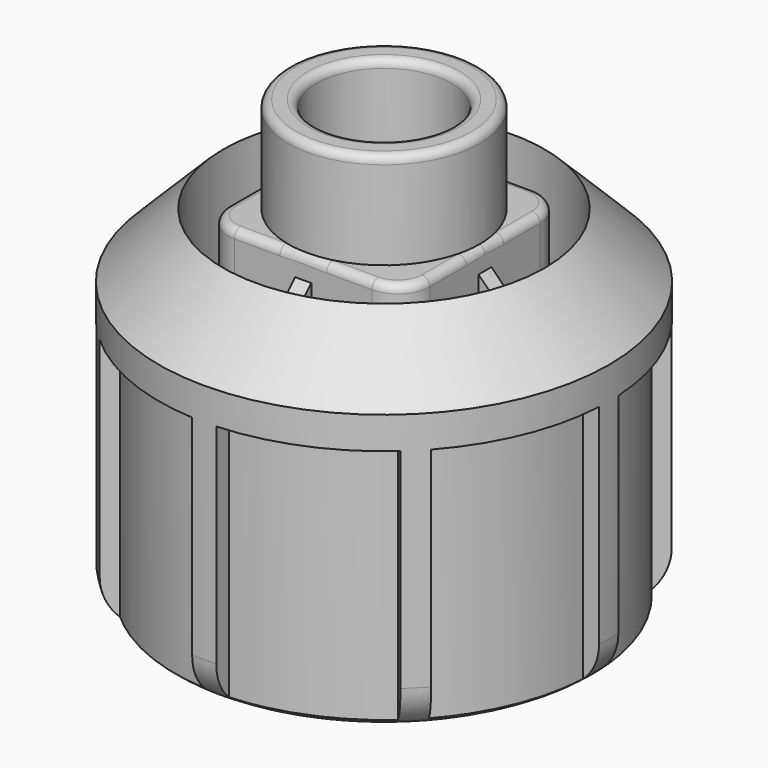
from build123d import *

# Parameters (mm, degrees)
F0_R          = 9.4615
F0_R_2        = 5.08
F1_DEPTH      = 44.45
F2_R          = 22.225
F2_R_2        = 5.08
F3_DEPTH      = 34.925
F4_R          = 6.6675
F5_DEPTH      = 8.128
F6_W          = 13.208
F6_H          = 13.208
F1_FACE1_R    = 9.4615
F1_FACE1_R_2  = 6.6675
F7_DEPTH      = 33.528
F8_R          = 15.875
F9_DEPTH      = 11.684
F10_W         = 3.175
F10_H         = 1.5875
F10_W_2       = 1.5875
F10_H_2       = 3.175
F11_DEPTH     = 9.525
F12_SIZE      = 3.17499
F14_DEPTH     = 25.4
F15_T2_ANGLE  = 33.7650687585
F15_T4_ANGLE  = 33.7650687585
F15_T6_ANGLE  = 67.5302236242
F15_T8_ANGLE  = 67.5302236242
F15_T10_ANGLE = 67.5302236242
F15_T12_ANGLE = 67.5302236242
F15_T14_ANGLE = 67.5302236242
F15_T16_ANGLE = 67.5302236242
F15_T18_ANGLE = 67.5302236242
F16_SIZE      = 6.34999
F17_R         = 0.79375


# Not quite as in the source:
# - a fillet or chamfer that OpenCascade refuses, or shapes differently, is made with other operations: its cross-section is extruded or revolved along the edge and cut away or added
# - a fillet or chamfer is up to 0.001 mm smaller than in the source, because OpenCascade refuses the exact size


with BuildPart() as f1:
    # F0 (on Top) → F1 (new body)
    with BuildSketch(Plane.XY):
        Circle(F0_R)
        Circle(F0_R_2, mode=Mode.SUBTRACT)
    extrude(amount=F1_DEPTH)

    # F2 (on face) → F3 (join)
    with BuildSketch(Plane(origin=(0, 0, 0), x_dir=(1, 0, 0), z_dir=(0, 0, -1))):
        Circle(F2_R)
        Circle(F2_R_2, mode=Mode.SUBTRACT)
    extrude(amount=-F3_DEPTH)

    # F4 (on face) → F5 (cut)
    with BuildSketch(Plane.XY.offset(44.45)):
        Circle(F4_R)
    extrude(amount=-F5_DEPTH, mode=Mode.SUBTRACT)

    # F6 (on face) + F1_face1 (on face) → F7 (cut)
    with BuildSketch(Plane(origin=(0, 0, 0), x_dir=(1, 0, 0), z_dir=(0, 0, -1))):
        Rectangle(F6_W, F6_H)
    with BuildSketch(Plane.XY.offset(44.45)):
        Circle(F1_FACE1_R)
        Circle(F1_FACE1_R_2, mode=Mode.SUBTRACT)
    extrude(amount=-F7_DEPTH, dir=(0, 0, -1), mode=Mode.SUBTRACT)

    # F8 (on face) → F9 (cut)
    with BuildSketch(Plane.XY.offset(34.925)):
        Circle(F8_R)
        with BuildLine():
            Line((-6.7945, 9.9695), (6.7945, 9.9695))
            ThreePointArc((6.7945, 9.9695), (9.0395640303, 9.0395640303), (9.9695, 6.7945))
            Line((9.9695, 6.7945), (9.9695, -6.7945))
            ThreePointArc((9.9695, -6.7945), (9.0395640303, -9.0395640303), (6.7945, -9.9695))
            Line((6.7945, -9.9695), (-6.7945, -9.9695))
            ThreePointArc((-6.7945, -9.9695), (-9.0395640303, -9.0395640303), (-9.9695, -6.7945))
            Line((-9.9695, -6.7945), (-9.9695, 6.7945))
            ThreePointArc((-9.9695, 6.7945), (-9.0395640303, 9.0395640303), (-6.7945, 9.9695))
        make_face(mode=Mode.SUBTRACT)
    extrude(amount=-F9_DEPTH, mode=Mode.SUBTRACT)

    # F10 (on face) → F11 (join)
    with BuildSketch(Plane.XY.offset(23.241)):
        with Locations((-11.557, 0)):
            Rectangle(F10_W, F10_H)
        with Locations((0, -11.557)):
            Rectangle(F10_W_2, F10_H_2)
        with Locations((11.557, 0)):
            Rectangle(F10_W, F10_H)
        with Locations((0, 11.557)):
            Rectangle(F10_W_2, F10_H_2)
    extrude(amount=F11_DEPTH)

    # F12 (size 3.175 in the source; OpenCascade refuses exactly that, so slightly less here)
    f12_edges = [f1.edges().sort_by_distance(p)[0] for p in [
        (-13.1445, 0, 32.766),
        (0, -13.1445, 32.766),
        (13.1445, 0, 32.766),
        (0, 13.1445, 32.766),
    ]]
    chamfer(f12_edges, length=F12_SIZE)

    # F13 (on face) → F14 (cut)
    with BuildSketch(Plane(origin=(0, 0, 0), x_dir=(1, 0, 0), z_dir=(0, 0, -1))):
        with BuildLine():
            Line((22.1930853445, -1.190625), (20.603126422, -1.190625))
            ThreePointArc((20.603126422, -1.190625), (19.0665638522, -7.8976293354), (15.410509418, -13.7267113953))
            Line((15.410509418, -13.7267113953), (16.5347801539, -14.8509821312))
            ThreePointArc((16.5347801539, -14.8509821312), (20.5332226101, -8.5051392843), (22.1930853445, -1.190625))
        make_face()
        with BuildLine():
            Line((14.8509821312, -16.5347801539), (13.7267113953, -15.410509418))
            ThreePointArc((13.7267113953, -15.410509418), (7.8976293354, -19.0665638522), (1.190625, -20.603126422))
            Line((1.190625, -20.603126422), (1.190625, -22.1930853445))
            ThreePointArc((1.190625, -22.1930853445), (8.5051392843, -20.5332226101), (14.8509821312, -16.5347801539))
        make_face()
        with BuildLine():
            Line((-1.190625, -22.1930853445), (-1.190625, -20.603126422))
            ThreePointArc((-1.190625, -20.603126422), (-7.8976293354, -19.0665638522), (-13.7267113953, -15.410509418))
            Line((-13.7267113953, -15.410509418), (-14.8509821312, -16.5347801539))
            ThreePointArc((-14.8509821312, -16.5347801539), (-8.5051392843, -20.5332226101), (-1.190625, -22.1930853445))
        make_face()
        with BuildLine():
            Line((-16.5347801539, -14.8509821312), (-15.410509418, -13.7267113953))
            ThreePointArc((-15.410509418, -13.7267113953), (-19.0665638522, -7.8976293354), (-20.603126422, -1.190625))
            Line((-20.603126422, -1.190625), (-22.1930853445, -1.190625))
            ThreePointArc((-22.1930853445, -1.190625), (-20.5332226101, -8.5051392843), (-16.5347801539, -14.8509821312))
        make_face()
        with BuildLine():
            ThreePointArc((-20.603126422, 1.190625), (-19.0665638522, 7.8976293354), (-15.410509418, 13.7267113953))
            Line((-15.410509418, 13.7267113953), (-16.5347801539, 14.8509821312))
            ThreePointArc((-16.5347801539, 14.8509821312), (-20.5332226101, 8.5051392843), (-22.1930853445, 1.190625))
            Line((-22.1930853445, 1.190625), (-20.603126422, 1.190625))
        make_face()
        with BuildLine():
            ThreePointArc((-13.7267113953, 15.410509418), (-7.8976293354, 19.0665638522), (-1.190625, 20.603126422))
            Line((-1.190625, 20.603126422), (-1.190625, 22.1930853445))
            ThreePointArc((-1.190625, 22.1930853445), (-8.5051392843, 20.5332226101), (-14.8509821312, 16.5347801539))
            Line((-14.8509821312, 16.5347801539), (-13.7267113953, 15.410509418))
        make_face()
        with BuildLine():
            ThreePointArc((1.190625, 20.603126422), (7.8976293354, 19.0665638522), (13.7267113953, 15.410509418))
            Line((13.7267113953, 15.410509418), (14.8509821312, 16.5347801539))
            ThreePointArc((14.8509821312, 16.5347801539), (8.5051392843, 20.5332226101), (1.190625, 22.1930853445))
            Line((1.190625, 22.1930853445), (1.190625, 20.603126422))
        make_face()
        with BuildLine():
            ThreePointArc((15.410509418, 13.7267113953), (19.0665638522, 7.8976293354), (20.603126422, 1.190625))
            Line((20.603126422, 1.190625), (22.1930853445, 1.190625))
            ThreePointArc((22.1930853445, 1.190625), (20.5332226101, 8.5051392843), (16.5347801539, 14.8509821312))
            Line((16.5347801539, 14.8509821312), (15.410509418, 13.7267113953))
        make_face()
    extrude(amount=-F14_DEPTH, mode=Mode.SUBTRACT)

    # F15: fillet of radius 4.7625 on 9 edges, made by hand

    # F15_s1 → F15_t2 (revolve, cut)
    with BuildSketch(Plane(origin=(0, 0, 0), x_dir=(0, 0, 1), z_dir=(-0.5557888899, 0.8313234689, 0))):
        with BuildLine():
            ThreePointArc((4.7625, 22.225), (1.3949039546, 20.8300960454), (0, 17.4625))
            Line((0, 17.4625), (0, 22.225))
            Line((0, 22.225), (4.7625, 22.225))
        make_face()
    revolve(axis=Axis((0, 0, 0), (0, 0, -1)), revolution_arc=F15_T2_ANGLE, mode=Mode.SUBTRACT)

    # F15_s3 → F15_t4 (revolve, cut)
    with BuildSketch(Plane.XZ):
        with BuildLine():
            ThreePointArc((22.225, 4.7625), (20.8300960454, 1.3949039546), (17.4625, 0))
            Line((17.4625, 0), (22.225, 0))
            Line((22.225, 0), (22.225, 4.7625))
        make_face()
    revolve(axis=Axis((0, 0, 0), (0, 0, -1)), revolution_arc=F15_T4_ANGLE, mode=Mode.SUBTRACT)

    # F15_s5 → F15_t6 (revolve, cut)
    with BuildSketch(Plane(origin=(0, 0, 0), x_dir=(0, 0, 1), z_dir=(0.1948316323, 0.9808367015, 0))):
        with BuildLine():
            ThreePointArc((4.7625, 22.225), (1.3949039546, 20.8300960454), (0, 17.4625))
            Line((0, 17.4625), (0, 22.225))
            Line((0, 22.225), (4.7625, 22.225))
        make_face()
    revolve(axis=Axis((0, 0, 0), (0, 0, -1)), revolution_arc=F15_T6_ANGLE, mode=Mode.SUBTRACT)

    # F15_s7 → F15_t8 (revolve, cut)
    with BuildSketch(Plane(origin=(0, 0, 0), x_dir=(0, 0, 1), z_dir=(0.8313230512, 0.5557895145, 0))):
        with BuildLine():
            ThreePointArc((4.7625, 22.225), (1.3949039546, 20.8300960454), (0, 17.4625))
            Line((0, 17.4625), (0, 22.225))
            Line((0, 22.225), (4.7625, 22.225))
        make_face()
    revolve(axis=Axis((0, 0, 0), (0, 0, -1)), revolution_arc=F15_T8_ANGLE, mode=Mode.SUBTRACT)

    # F15_s9 → F15_t10 (revolve, cut)
    with BuildSketch(Plane(origin=(0, 0, 0), x_dir=(0, 0, 1), z_dir=(0.9808367015, -0.1948316323, 0))):
        with BuildLine():
            ThreePointArc((4.7625, 22.225), (1.3949039546, 20.8300960454), (0, 17.4625))
            Line((0, 17.4625), (0, 22.225))
            Line((0, 22.225), (4.7625, 22.225))
        make_face()
    revolve(axis=Axis((0, 0, 0), (0, 0, -1)), revolution_arc=F15_T10_ANGLE, mode=Mode.SUBTRACT)

    # F15_s11 → F15_t12 (revolve, cut)
    with BuildSketch(Plane(origin=(0, 0, 0), x_dir=(0, 0, 1), z_dir=(0.5557895145, -0.8313230512, 0))):
        with BuildLine():
            ThreePointArc((4.7625, 22.225), (1.3949039546, 20.8300960454), (0, 17.4625))
            Line((0, 17.4625), (0, 22.225))
            Line((0, 22.225), (4.7625, 22.225))
        make_face()
    revolve(axis=Axis((0, 0, 0), (0, 0, -1)), revolution_arc=F15_T12_ANGLE, mode=Mode.SUBTRACT)

    # F15_s13 → F15_t14 (revolve, cut)
    with BuildSketch(Plane(origin=(0, 0, 0), x_dir=(0, 0, 1), z_dir=(-0.1948316323, -0.9808367015, 0))):
        with BuildLine():
            ThreePointArc((4.7625, 22.225), (1.3949039546, 20.8300960454), (0, 17.4625))
            Line((0, 17.4625), (0, 22.225))
            Line((0, 22.225), (4.7625, 22.225))
        make_face()
    revolve(axis=Axis((0, 0, 0), (0, 0, -1)), revolution_arc=F15_T14_ANGLE, mode=Mode.SUBTRACT)

    # F15_s15 → F15_t16 (revolve, cut)
    with BuildSketch(Plane(origin=(0, 0, 0), x_dir=(0, 0, 1), z_dir=(-0.8313230512, -0.5557895145, 0))):
        with BuildLine():
            ThreePointArc((4.7625, 22.225), (1.3949039546, 20.8300960454), (0, 17.4625))
            Line((0, 17.4625), (0, 22.225))
            Line((0, 22.225), (4.7625, 22.225))
        make_face()
    revolve(axis=Axis((0, 0, 0), (0, 0, -1)), revolution_arc=F15_T16_ANGLE, mode=Mode.SUBTRACT)

    # F15_s17 → F15_t18 (revolve, cut)
    with BuildSketch(Plane(origin=(0, 0, 0), x_dir=(0, 0, 1), z_dir=(-0.9808367015, 0.1948316323, 0))):
        with BuildLine():
            ThreePointArc((4.7625, 22.225), (1.3949039546, 20.8300960454), (0, 17.4625))
            Line((0, 17.4625), (0, 22.225))
            Line((0, 22.225), (4.7625, 22.225))
        make_face()
    revolve(axis=Axis((0, 0, 0), (0, 0, -1)), revolution_arc=F15_T18_ANGLE, mode=Mode.SUBTRACT)

    # F16 (size 6.35 in the source; OpenCascade refuses exactly that, so slightly less here)
    f16_edges = [f1.edges().sort_by_distance(p)[0] for p in [
        (-22.225, 0, 34.925),
    ]]
    chamfer(f16_edges, length=F16_SIZE)

    # F17
    f17_edges = [f1.edges().sort_by_distance(p)[0] for p in [
        (0, 9.9695, 34.925),
        (-9.4615, 0, 44.45),
        (-6.6675, 0, 44.45),
        (-9.039564, 9.039564, 34.925),
        (-9.039564, -9.039564, 34.925),
        (9.039564, -9.039564, 34.925),
        (9.039564, 9.039564, 34.925),
    ]]
    fillet(f17_edges, radius=F17_R)


solid = f1.part
